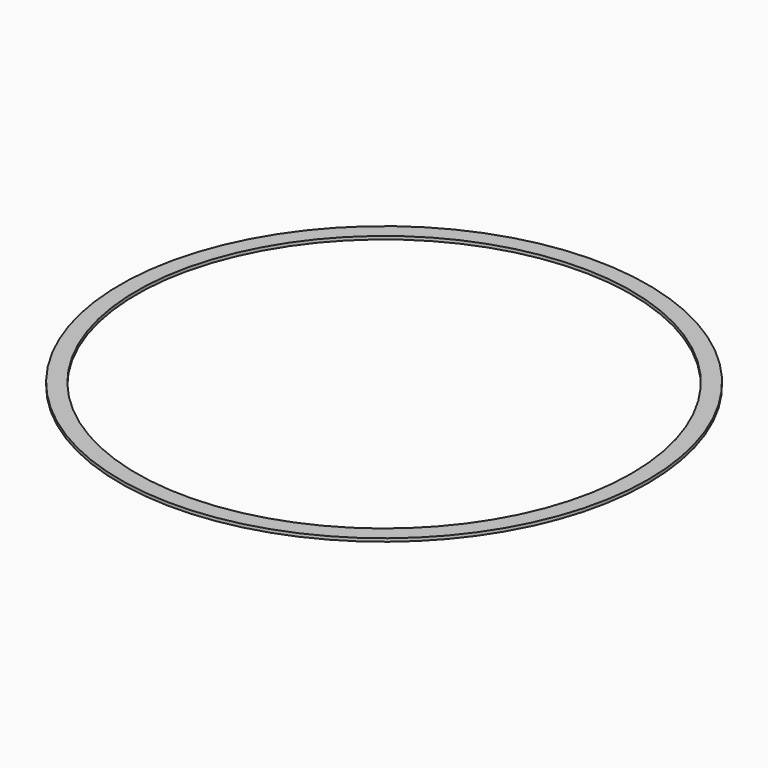
from build123d import *

# Parameters (mm, degrees)
F0_R     = 404.02002
F0_R_2   = 378.62002
F1_DEPTH = 4.7625


# Not quite as in the source:
# - a length typed as a fraction of an inch, garbled in the dataset ("3 / 203.2 mm" for 3/8 in), is restored


with BuildPart() as f1:
    # F0 (on Top) → F1 (new body)
    with BuildSketch(Plane.XY):
        Circle(F0_R)
        Circle(F0_R_2, mode=Mode.SUBTRACT)
    extrude(amount=F1_DEPTH)


solid = f1.part
